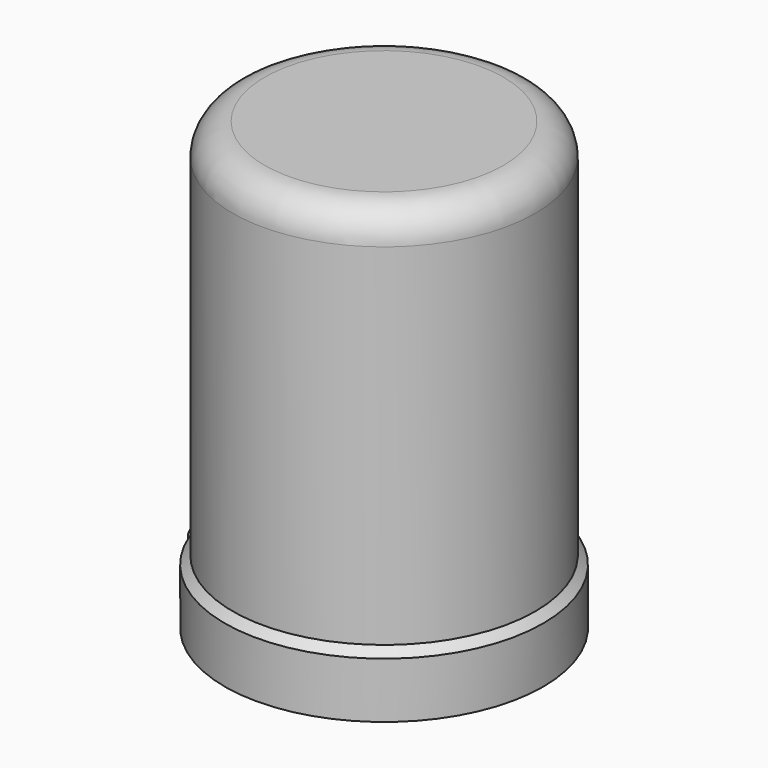
from build123d import *

# Parameters (mm, degrees)
F0_R     = 50
F1_DEPTH = 20
F2_R     = 47.5
F3_DEPTH = 120
F4_R     = 10
F5_SIZE  = 2.49999
F7_DEPTH = 13
F8_R     = 2
F9_DEPTH = 5


# Not quite as in the source:
# - a fillet or chamfer is up to 0.001 mm smaller than in the source, because OpenCascade refuses the exact size


with BuildPart() as f1:
    # F0 (on Top) → F1 (new body)
    with BuildSketch(Plane.XY):
        Circle(F0_R)
    extrude(amount=F1_DEPTH)

    # F2 (on face) → F3 (join)
    with BuildSketch(Plane.XY.offset(20)):
        Circle(F2_R)
    extrude(amount=F3_DEPTH)

    # F4
    f4_edges = [f1.edges().sort_by_distance(p)[0] for p in [
        (-47.5, 0, 140),
    ]]
    fillet(f4_edges, radius=F4_R)

    # F5 (size 2.5 in the source; OpenCascade refuses exactly that, so slightly less here)
    f5_edges = [f1.edges().sort_by_distance(p)[0] for p in [
        (-50, 0, 20),
    ]]
    chamfer(f5_edges, length=F5_SIZE)

    # F6 (on face) → F7 (join)
    with BuildSketch(Plane(origin=(0, 0, 0), x_dir=(1, 0, 0), z_dir=(0, 0, -1))):
        with BuildLine():
            Line((-50, 0), (-55, 0))
            Line((-55, 0), (-55, -5))
            Line((-55, -5), (-49.7493718553, -5))
            ThreePointArc((-49.7493718553, -5), (-49.9373036555, -2.503138753), (-50, 0))
        make_face()
        with BuildLine():
            Line((-55, 5), (-55, 0))
            Line((-55, 0), (-50, 0))
            ThreePointArc((-50, 0), (-49.9373036555, 2.503138753), (-49.7493718553, 5))
            Line((-49.7493718553, 5), (-55, 5))
        make_face()
    extrude(amount=-F7_DEPTH)

    # F8 (on face) → F9 (join)
    with BuildSketch(Plane(origin=(-55, 0, 0), x_dir=(0, -1, 0), z_dir=(-1, 0, 0))):
        with Locations((0, 6.5)):
            Circle(F8_R)
    extrude(amount=F9_DEPTH)


solid = f1.part
